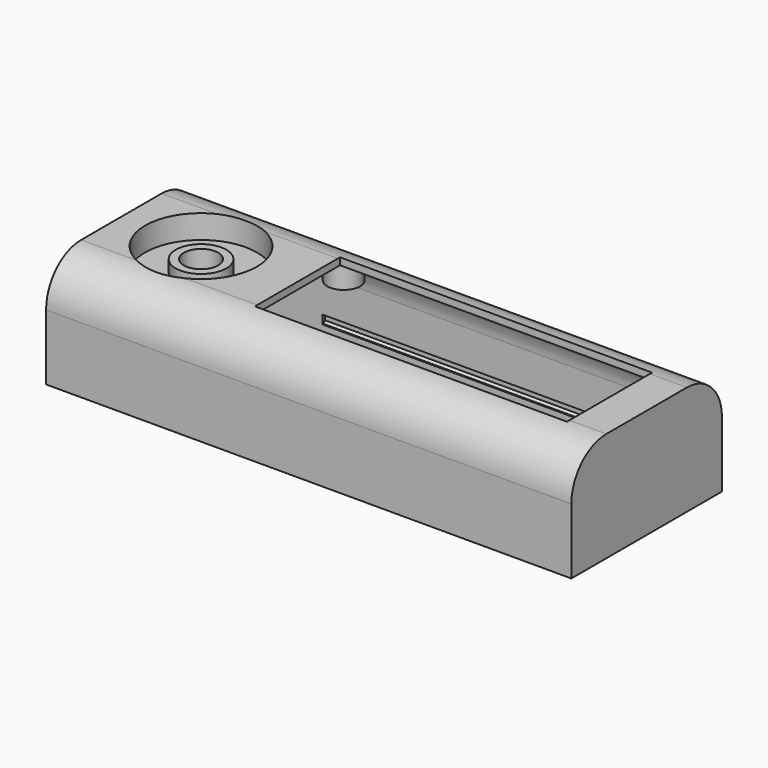
from build123d import *

# Parameters (mm, degrees)
F1_DEPTH  = 60
F2_T      = -1.6
F4_R      = 3.75
F4_R_2    = 1.25
F4_R_3    = 3.65
F4_R_4    = 3.25
F4_R_5    = 12.75
F4_W      = 71.3
F4_H      = 24.3
F6_DEPTH  = 6.601
F4_R_6    = 13.95
F7_DEPTH  = 1.2
F8_R      = 3.925
F9_DEPTH  = 6.6010001
F8_R_2    = 5.775
F10_DEPTH = 4
F11_DEPTH = 5
F12_W     = 60
F12_H     = 2
F13_DEPTH = 0.8
F14_SIZE  = 0.5


with BuildPart() as f1:
    # F0 (on Right) → F1 (new body, symmetric)
    with BuildSketch(Plane.YZ):
        with BuildLine():
            Line((-21.5, 15), (-21.5, 0))
            Line((-21.5, 0), (21.5, 0))
            Line((21.5, 0), (21.5, 15))
            ThreePointArc((21.5, 15), (18.5710678119, 22.0710678119), (11.5, 25))
            Line((11.5, 25), (-11.5, 25))
            ThreePointArc((-11.5, 25), (-18.5710678119, 22.0710678119), (-21.5, 15))
        make_face()
    extrude(amount=F1_DEPTH, both=True)

    # F2
    f2_openings = [f1.faces().sort_by_distance(p)[0] for p in [
        (0, 0, 0),
    ]]
    offset(amount=F2_T, openings=f2_openings)

    # F4 (on offset) → F5 (join, up to the next surface of F1)
    with BuildSketch(Plane(origin=(0, 0, 18.4), x_dir=(1, 0, 0), z_dir=(0, 0, -1))):
        with Locations((53.4, -15.5)):
            Circle(F4_R)
        with Locations((53.4, -15.5)):
            Circle(F4_R_2, mode=Mode.SUBTRACT)
        with Locations((53.4, 15.5)):
            Circle(F4_R_3)
        with Locations((53.4, 15.5)):
            Circle(F4_R_2, mode=Mode.SUBTRACT)
        with Locations((-21.6, -15.5)):
            Circle(F4_R)
        with Locations((-21.6, -15.5)):
            Circle(F4_R_2, mode=Mode.SUBTRACT)
        with Locations((-21.6, 15.5)):
            Circle(F4_R_4)
        with Locations((-21.6, 15.5)):
            Circle(F4_R_2, mode=Mode.SUBTRACT)
    extrude(until=Until.NEXT, dir=(0, 0, 1))

    # F4 (on offset) → F6 (cut, through all)
    with BuildSketch(Plane(origin=(0, 0, 18.4), x_dir=(1, 0, 0), z_dir=(0, 0, -1))):
        with Locations((-41.8, 0)):
            Circle(F4_R_5)
        with Locations((15.9, 0)):
            Rectangle(F4_W, F4_H)
    extrude(amount=-F6_DEPTH, mode=Mode.SUBTRACT)



with BuildPart() as f7:
    # F4 (on offset) → F7 (new body)
    with BuildSketch(Plane(origin=(0, 0, 18.4), x_dir=(1, 0, 0), z_dir=(0, 0, -1))):
        with Locations((-41.8, 0)):
            Circle(F4_R_6)
        with Locations((-41.8, 0)):
            Circle(F4_R_5, mode=Mode.SUBTRACT)
        with Locations((-41.8, 0)):
            Circle(F4_R_5)
    extrude(amount=-F7_DEPTH)

    # F8 (on face) → F9 (cut, through all)
    with BuildSketch(Plane(origin=(0, 0, 18.4), x_dir=(1, 0, 0), z_dir=(0, 0, -1))):
        with Locations((-41.8, 0)):
            Circle(F8_R)
    extrude(amount=-F9_DEPTH, mode=Mode.SUBTRACT)

    # F8 (on face) → F10 (join)
    with BuildSketch(Plane(origin=(0, 0, 18.4), x_dir=(1, 0, 0), z_dir=(0, 0, -1))):
        with Locations((-41.8, 0)):
            Circle(F8_R_2)
        with Locations((-41.8, 0)):
            Circle(F8_R, mode=Mode.SUBTRACT)
    extrude(amount=-F10_DEPTH)


with BuildPart() as f1_1:
    add(f1.part)

    add(f7.part)  # F11 merges F7
    # F4 (on offset) → F11 (join, through all)
    with BuildSketch(Plane(origin=(0, 0, 18.4), x_dir=(1, 0, 0), z_dir=(0, 0, -1))):
        with Locations((-41.8, 0)):
            Circle(F4_R_6)
        with Locations((-41.8, 0)):
            Circle(F4_R_5, mode=Mode.SUBTRACT)
    extrude(amount=-F11_DEPTH)


with BuildPart() as f13:
    # F12 (on face) → F13 (new body)
    with BuildSketch(Plane.XZ.offset(-19.9)):
        with Locations((0, 6)):
            Rectangle(F12_W, F12_H)
    extrude(amount=-F13_DEPTH)

    # F14
    f14_edges = [f13.edges().sort_by_distance(p)[0] for p in [
        (0, 20.7, 5),
        (0, 20.7, 7),
    ]]
    chamfer(f14_edges, length=F14_SIZE)


with BuildPart() as f15_1:
    # F15: instance of F13
    add(f13.part.mirror(Plane.XZ))


with BuildPart() as f1_2:
    add(f1_1.part)

    # F16: cut F13, F15_1
    add(f13.part, mode=Mode.SUBTRACT)
    add(f15_1.part, mode=Mode.SUBTRACT)


solid = f1_2.part
